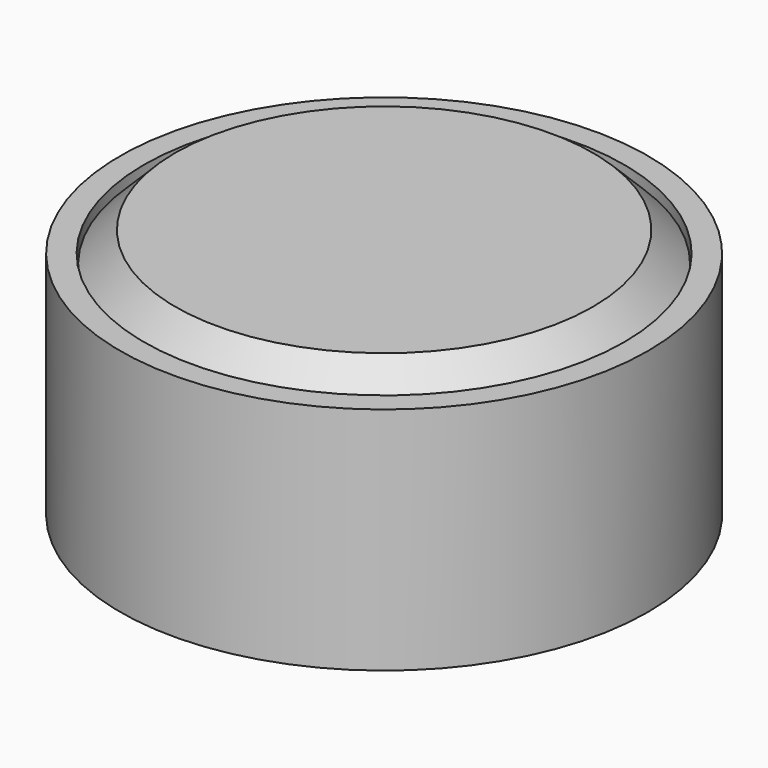
from build123d import *

# Parameters (mm, degrees)
F2_R      = 20.06694
F3_DEPTH  = 19.05
F5_R      = 5.0538
F6_DEPTH  = 4.793996
F7_COUNT  = 9
F9_SIZE   = 2.54
F10_R     = 22.16694
F10_R_2   = 20.16694
F11_DEPTH = 19.304


# Not quite as in the source:
# - a feature names something its author has since deleted; it is built from what else it names


with BuildPart() as f1:
    # F0 (on Front) → F1 (revolve)
    with BuildSketch(Plane.XZ):
        Polygon((0, 21.05), (0, 19.05), (14.478, 19.05), (14.478, 0), (20.06694, 0), (20.06694, 21.05), align=None)
    revolve(axis=Axis((0, 0, 5.8315382339), (0, 0, 1)))

    # F2 (on face) → F3 (join, through all)
    with BuildSketch(Plane(origin=(0, 0, 0), x_dir=(1, 0, 0), z_dir=(0, 0, -1))):
        Circle(F2_R)
        with BuildLine():
            ThreePointArc((1.3953731968, 14.4106008772), (10.237491978, 10.237491978), (14.4106008772, 1.3953731968))
            ThreePointArc((14.4106008772, 1.3953731968), (15.4417044219, 1.0113766792), (15.875, 0))
            ThreePointArc((15.875, 0), (15.4417044219, -1.0113766792), (14.4106008772, -1.3953731968))
            ThreePointArc((14.4106008772, -1.3953731968), (10.237491978, -10.237491978), (1.3953731968, -14.4106008772))
            ThreePointArc((1.3953731968, -14.4106008772), (1.39659324, -14.4442906235), (1.397, -14.478))
            ThreePointArc((1.397, -14.478), (-0.0337093765, -15.87459324), (-1.3953731968, -14.4106008772))
            ThreePointArc((-1.3953731968, -14.4106008772), (-10.237491978, -10.237491978), (-14.4106008772, -1.3953731968))
            ThreePointArc((-14.4106008772, -1.3953731968), (-15.875, 0), (-14.4106008772, 1.3953731968))
            ThreePointArc((-14.4106008772, 1.3953731968), (-10.237491978, 10.237491978), (-1.3953731968, 14.4106008772))
            ThreePointArc((-1.3953731968, 14.4106008772), (-0.0337093765, 15.87459324), (1.397, 14.478))
            ThreePointArc((1.397, 14.478), (1.39659324, 14.4442906235), (1.3953731968, 14.4106008772))
        make_face(mode=Mode.SUBTRACT)
        with BuildLine():
            ThreePointArc((-1.3953731968, 14.4106008772), (0, 13.081), (1.3953731968, 14.4106008772))
            ThreePointArc((1.3953731968, 14.4106008772), (0, 14.478), (-1.3953731968, 14.4106008772))
        make_face()
        with BuildLine():
            ThreePointArc((14.4106008772, -1.3953731968), (14.4611404028, -0.6985), (14.478, 0))
            ThreePointArc((14.478, 0), (14.4611404028, 0.6985), (14.4106008772, 1.3953731968))
            ThreePointArc((14.4106008772, 1.3953731968), (13.081, 0), (14.4106008772, -1.3953731968))
        make_face()
        with BuildLine():
            ThreePointArc((14.4106008772, 1.3953731968), (14.4611404028, 0.6985), (14.478, 0))
            ThreePointArc((14.478, 0), (14.4611404028, -0.6985), (14.4106008772, -1.3953731968))
            ThreePointArc((14.4106008772, -1.3953731968), (15.4417044219, -1.0113766792), (15.875, 0))
            ThreePointArc((15.875, 0), (15.4417044219, 1.0113766792), (14.4106008772, 1.3953731968))
        make_face()
        with BuildLine():
            ThreePointArc((-1.3953731968, -14.4106008772), (0, -14.478), (1.3953731968, -14.4106008772))
            ThreePointArc((1.3953731968, -14.4106008772), (0, -13.081), (-1.3953731968, -14.4106008772))
        make_face()
        with BuildLine():
            ThreePointArc((1.397, -14.478), (1.39659324, -14.4442906235), (1.3953731968, -14.4106008772))
            ThreePointArc((1.3953731968, -14.4106008772), (0, -14.478), (-1.3953731968, -14.4106008772))
            ThreePointArc((-1.3953731968, -14.4106008772), (-0.0337093765, -15.87459324), (1.397, -14.478))
        make_face()
        with BuildLine():
            ThreePointArc((-14.4106008772, -1.3953731968), (-14.478, 0), (-14.4106008772, 1.3953731968))
            ThreePointArc((-14.4106008772, 1.3953731968), (-15.875, 0), (-14.4106008772, -1.3953731968))
        make_face()
        with BuildLine():
            ThreePointArc((-13.081, 0), (-13.4666233208, 0.9637044219), (-14.4106008772, 1.3953731968))
            ThreePointArc((-14.4106008772, 1.3953731968), (-14.478, 0), (-14.4106008772, -1.3953731968))
            ThreePointArc((-14.4106008772, -1.3953731968), (-13.4666233208, -0.9637044219), (-13.081, 0))
        make_face()
    extrude(amount=-F3_DEPTH)


with BuildPart() as f6:
    # F5 (on offset) → F6 (new body)
    with BuildSketch(Plane.YZ.offset(20.0669398)):
        with Locations((0, 10.525)):
            Circle(F5_R)
    extrude(amount=-F6_DEPTH)


with BuildPart() as f7_1:
    # F7: instance of F6
    add(f6.part.rotate(Axis((0, 0, 5.8315382339), (0, 0, 1)), 1 * 360 / F7_COUNT))


with BuildPart() as f7_2:
    # F7: instance of F6
    add(f6.part.rotate(Axis((0, 0, 5.8315382339), (0, 0, 1)), 2 * 360 / F7_COUNT))


with BuildPart() as f7_3:
    # F7: instance of F6
    add(f6.part.rotate(Axis((0, 0, 5.8315382339), (0, 0, 1)), 3 * 360 / F7_COUNT))


with BuildPart() as f7_4:
    # F7: instance of F6
    add(f6.part.rotate(Axis((0, 0, 5.8315382339), (0, 0, 1)), 4 * 360 / F7_COUNT))


with BuildPart() as f7_5:
    # F7: instance of F6
    add(f6.part.rotate(Axis((0, 0, 5.8315382339), (0, 0, 1)), 5 * 360 / F7_COUNT))


with BuildPart() as f7_6:
    # F7: instance of F6
    add(f6.part.rotate(Axis((0, 0, 5.8315382339), (0, 0, 1)), 6 * 360 / F7_COUNT))


with BuildPart() as f7_7:
    # F7: instance of F6
    add(f6.part.rotate(Axis((0, 0, 5.8315382339), (0, 0, 1)), 7 * 360 / F7_COUNT))


with BuildPart() as f7_8:
    # F7: instance of F6
    add(f6.part.rotate(Axis((0, 0, 5.8315382339), (0, 0, 1)), 8 * 360 / F7_COUNT))


with BuildPart() as f1_1:
    add(f1.part)

    # F8: cut F6, F7_2, F7_4, F7_6, F7_8, F7_7, F7_5, F7_3, F7_1
    add(f6.part, mode=Mode.SUBTRACT)
    add(f7_2.part, mode=Mode.SUBTRACT)
    add(f7_4.part, mode=Mode.SUBTRACT)
    add(f7_6.part, mode=Mode.SUBTRACT)
    add(f7_8.part, mode=Mode.SUBTRACT)
    add(f7_7.part, mode=Mode.SUBTRACT)
    add(f7_5.part, mode=Mode.SUBTRACT)
    add(f7_3.part, mode=Mode.SUBTRACT)
    add(f7_1.part, mode=Mode.SUBTRACT)

    # F9
    f9_edges = [f1_1.edges().sort_by_distance(p)[0] for p in [
        (-20.06694, 0, 21.05),
    ]]
    chamfer(f9_edges, length=F9_SIZE)


with BuildPart() as f11:
    # F10 (on face) → F11 (new body)
    with BuildSketch(Plane(origin=(0, 0, 0), x_dir=(1, 0, 0), z_dir=(0, 0, -1))):
        Circle(F10_R)
        Circle(F10_R_2, mode=Mode.SUBTRACT)
    extrude(amount=-F11_DEPTH)


solid = Compound([f1_1.part, f11.part])
